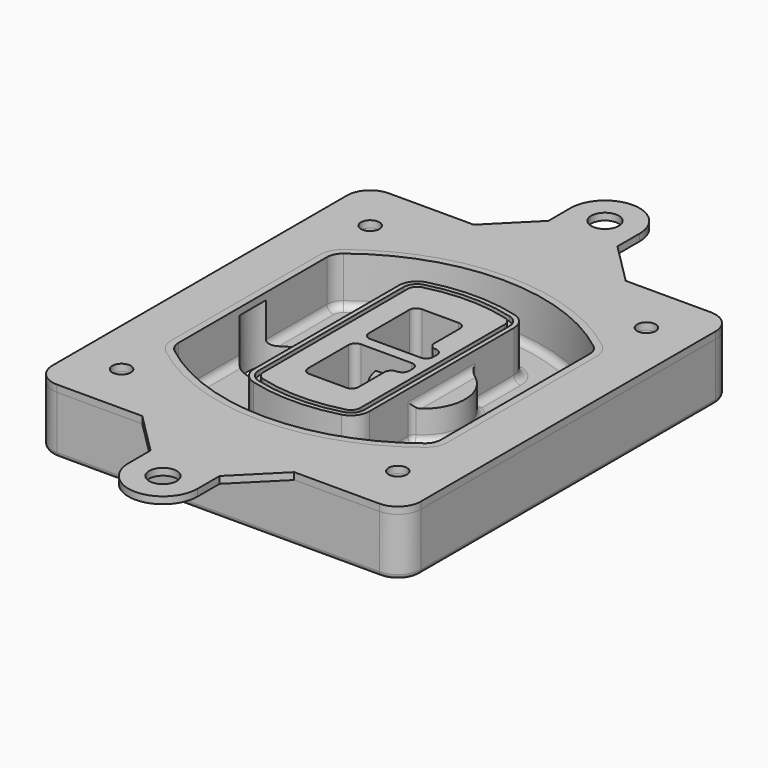
from build123d import *

# Parameters (mm, degrees)
F0_R      = 4
F1_DEPTH  = 25
F2_DEPTH  = 3
F3_DEPTH  = 18
F5_DEPTH  = 21
F6_DEPTH  = 2
F8_DEPTH  = 20
F9_DEPTH  = 16
F10_DEPTH = 25
F7_R      = 6
F7_R_2    = 4
F11_DEPTH = 6
F13_DEPTH = 9
F14_R     = 3
F15_R     = 2
F16_R     = 6
F16_R_2   = 4
F17_DEPTH = 3


with BuildPart() as f1:
    # F0 (on Top) → F1 (new body)
    with BuildSketch(Plane.XY):
        with BuildLine():
            ThreePointArc((-80, -80), (-77.0710678119, -87.0710678119), (-70, -90))
            Line((-70, -90), (70, -90))
            ThreePointArc((70, -90), (77.0710678119, -87.0710678119), (80, -80))
            Line((80, -80), (80, 80))
            ThreePointArc((80, 80), (77.0710678119, 87.0710678119), (70, 90))
            Line((70, 90), (-70, 90))
            ThreePointArc((-70, 90), (-77.0710678119, 87.0710678119), (-80, 80))
            Line((-80, 80), (-80, -80))
        make_face()
        with Locations((-60, -67.5)):
            Circle(F0_R, mode=Mode.SUBTRACT)
        with Locations((60, -67.5)):
            Circle(F0_R, mode=Mode.SUBTRACT)
        with Locations((-60, 67.5)):
            Circle(F0_R, mode=Mode.SUBTRACT)
        with BuildLine():
            ThreePointArc((-64, 40.2934422872), (-62.5820384798, 46.4328484224), (-58.6153846154, 51.3286200352))
            ThreePointArc((-58.6153846154, 51.3286200352), (0, 71.5), (58.6153846154, 51.3286200352))
            ThreePointArc((58.6153846154, 51.3286200352), (62.5820384798, 46.4328484224), (64, 40.2934422872))
            Line((64, 40.2934422872), (64, -40.2934422872))
            ThreePointArc((64, -40.2934422872), (62.5820384798, -46.4328484224), (58.6153846154, -51.3286200352))
            ThreePointArc((58.6153846154, -51.3286200352), (0, -71.5), (-58.6153846154, -51.3286200352))
            ThreePointArc((-58.6153846154, -51.3286200352), (-62.5820384798, -46.4328484224), (-64, -40.2934422872))
            Line((-64, -40.2934422872), (-64, 40.2934422872))
        make_face(mode=Mode.SUBTRACT)
        with Locations((60, 67.5)):
            Circle(F0_R, mode=Mode.SUBTRACT)
        with BuildLine():
            ThreePointArc((58.6153846154, 51.3286200352), (0, 71.5), (-58.6153846154, 51.3286200352))
            ThreePointArc((-58.6153846154, 51.3286200352), (-62.5820384798, 46.4328484224), (-64, 40.2934422872))
            Line((-64, 40.2934422872), (-64, -40.2934422872))
            ThreePointArc((-64, -40.2934422872), (-62.5820384798, -46.4328484224), (-58.6153846154, -51.3286200352))
            ThreePointArc((-58.6153846154, -51.3286200352), (0, -71.5), (58.6153846154, -51.3286200352))
            ThreePointArc((58.6153846154, -51.3286200352), (62.5820384798, -46.4328484224), (64, -40.2934422872))
            Line((64, -40.2934422872), (64, 40.2934422872))
            ThreePointArc((64, 40.2934422872), (62.5820384798, 46.4328484224), (58.6153846154, 51.3286200352))
        make_face()
        with BuildLine():
            Line((-60, -40.2934422872), (-60, 40.2934422872))
            ThreePointArc((-60, 40.2934422872), (-58.9871703427, 44.6787323838), (-56.1538461538, 48.1757121072))
            ThreePointArc((-56.1538461538, 48.1757121072), (0, 67.5), (56.1538461538, 48.1757121072))
            ThreePointArc((56.1538461538, 48.1757121072), (58.9871703427, 44.6787323838), (60, 40.2934422872))
            Line((60, 40.2934422872), (60, -40.2934422872))
            ThreePointArc((60, -40.2934422872), (58.9871703427, -44.6787323838), (56.1538461538, -48.1757121072))
            ThreePointArc((56.1538461538, -48.1757121072), (0, -67.5), (-56.1538461538, -48.1757121072))
            ThreePointArc((-56.1538461538, -48.1757121072), (-58.9871703427, -44.6787323838), (-60, -40.2934422872))
        make_face(mode=Mode.SUBTRACT)
        with BuildLine():
            ThreePointArc((-56.1538461538, 48.1757121072), (-58.9871703427, 44.6787323838), (-60, 40.2934422872))
            Line((-60, 40.2934422872), (-60, -40.2934422872))
            ThreePointArc((-60, -40.2934422872), (-58.9871703427, -44.6787323838), (-56.1538461538, -48.1757121072))
            ThreePointArc((-56.1538461538, -48.1757121072), (0, -67.5), (56.1538461538, -48.1757121072))
            ThreePointArc((56.1538461538, -48.1757121072), (58.9871703427, -44.6787323838), (60, -40.2934422872))
            Line((60, -40.2934422872), (60, 40.2934422872))
            ThreePointArc((60, 40.2934422872), (58.9871703427, 44.6787323838), (56.1538461538, 48.1757121072))
            ThreePointArc((56.1538461538, 48.1757121072), (0, 67.5), (-56.1538461538, 48.1757121072))
        make_face()
        with BuildLine():
            ThreePointArc((54.3076923077, 45.8110311612), (56.2910192399, 43.3631453548), (57, 40.2934422872))
            Line((57, 40.2934422872), (57, -40.2934422872))
            ThreePointArc((57, -40.2934422872), (56.2910192399, -43.3631453548), (54.3076923077, -45.8110311612))
            ThreePointArc((54.3076923077, -45.8110311612), (0, -64.5), (-54.3076923077, -45.8110311612))
            ThreePointArc((-54.3076923077, -45.8110311612), (-56.2910192399, -43.3631453548), (-57, -40.2934422872))
            Line((-57, -40.2934422872), (-57, 40.2934422872))
            ThreePointArc((-57, 40.2934422872), (-56.2910192399, 43.3631453548), (-54.3076923077, 45.8110311612))
            ThreePointArc((-54.3076923077, 45.8110311612), (0, 64.5), (54.3076923077, 45.8110311612))
        make_face(mode=Mode.SUBTRACT)
        with BuildLine():
            Line((57, -40.2934422872), (57, 40.2934422872))
            ThreePointArc((57, 40.2934422872), (56.2910192399, 43.3631453548), (54.3076923077, 45.8110311612))
            ThreePointArc((54.3076923077, 45.8110311612), (0, 64.5), (-54.3076923077, 45.8110311612))
            ThreePointArc((-54.3076923077, 45.8110311612), (-56.2910192399, 43.3631453548), (-57, 40.2934422872))
            Line((-57, 40.2934422872), (-57, -40.2934422872))
            ThreePointArc((-57, -40.2934422872), (-56.2910192399, -43.3631453548), (-54.3076923077, -45.8110311612))
            ThreePointArc((-54.3076923077, -45.8110311612), (0, -64.5), (54.3076923077, -45.8110311612))
            ThreePointArc((54.3076923077, -45.8110311612), (56.2910192399, -43.3631453548), (57, -40.2934422872))
        make_face()
    extrude(amount=-F1_DEPTH)

    # F0 (on Top) → F2 (join)
    with BuildSketch(Plane.XY):
        with BuildLine():
            ThreePointArc((-56.1538461538, 48.1757121072), (-58.9871703427, 44.6787323838), (-60, 40.2934422872))
            Line((-60, 40.2934422872), (-60, -40.2934422872))
            ThreePointArc((-60, -40.2934422872), (-58.9871703427, -44.6787323838), (-56.1538461538, -48.1757121072))
            ThreePointArc((-56.1538461538, -48.1757121072), (0, -67.5), (56.1538461538, -48.1757121072))
            ThreePointArc((56.1538461538, -48.1757121072), (58.9871703427, -44.6787323838), (60, -40.2934422872))
            Line((60, -40.2934422872), (60, 40.2934422872))
            ThreePointArc((60, 40.2934422872), (58.9871703427, 44.6787323838), (56.1538461538, 48.1757121072))
            ThreePointArc((56.1538461538, 48.1757121072), (0, 67.5), (-56.1538461538, 48.1757121072))
        make_face()
        with BuildLine():
            ThreePointArc((54.3076923077, 45.8110311612), (56.2910192399, 43.3631453548), (57, 40.2934422872))
            Line((57, 40.2934422872), (57, -40.2934422872))
            ThreePointArc((57, -40.2934422872), (56.2910192399, -43.3631453548), (54.3076923077, -45.8110311612))
            ThreePointArc((54.3076923077, -45.8110311612), (0, -64.5), (-54.3076923077, -45.8110311612))
            ThreePointArc((-54.3076923077, -45.8110311612), (-56.2910192399, -43.3631453548), (-57, -40.2934422872))
            Line((-57, -40.2934422872), (-57, 40.2934422872))
            ThreePointArc((-57, 40.2934422872), (-56.2910192399, 43.3631453548), (-54.3076923077, 45.8110311612))
            ThreePointArc((-54.3076923077, 45.8110311612), (0, 64.5), (54.3076923077, 45.8110311612))
        make_face(mode=Mode.SUBTRACT)
    extrude(amount=F2_DEPTH)

    # F0 (on Top) → F3 (cut)
    with BuildSketch(Plane.XY):
        with BuildLine():
            Line((57, -40.2934422872), (57, 40.2934422872))
            ThreePointArc((57, 40.2934422872), (56.2910192399, 43.3631453548), (54.3076923077, 45.8110311612))
            ThreePointArc((54.3076923077, 45.8110311612), (0, 64.5), (-54.3076923077, 45.8110311612))
            ThreePointArc((-54.3076923077, 45.8110311612), (-56.2910192399, 43.3631453548), (-57, 40.2934422872))
            Line((-57, 40.2934422872), (-57, -40.2934422872))
            ThreePointArc((-57, -40.2934422872), (-56.2910192399, -43.3631453548), (-54.3076923077, -45.8110311612))
            ThreePointArc((-54.3076923077, -45.8110311612), (0, -64.5), (54.3076923077, -45.8110311612))
            ThreePointArc((54.3076923077, -45.8110311612), (56.2910192399, -43.3631453548), (57, -40.2934422872))
        make_face()
    extrude(amount=-F3_DEPTH, mode=Mode.SUBTRACT)

    # F4 (on face) → F5 (join, through all)
    with BuildSketch(Plane.XY.offset(3)):
        with BuildLine():
            ThreePointArc((-25, -39.2465276821), (-23.3511545998, -44.1109737193), (-19.0842911877, -46.9702398883))
            ThreePointArc((-19.0842911877, -46.9702398883), (0, -49.5), (19.0842911877, -46.9702398883))
            ThreePointArc((19.0842911877, -46.9702398883), (23.3511545998, -44.1109737193), (25, -39.2465276821))
            Line((25, -39.2465276821), (25, 39.2465276821))
            ThreePointArc((25, 39.2465276821), (23.3511545998, 44.1109737193), (19.0842911877, 46.9702398883))
            ThreePointArc((19.0842911877, 46.9702398883), (0, 49.5), (-19.0842911877, 46.9702398883))
            ThreePointArc((-19.0842911877, 46.9702398883), (-23.3511545998, 44.1109737193), (-25, 39.2465276821))
            Line((-25, 39.2465276821), (-25, -39.2465276821))
        make_face()
        with BuildLine():
            ThreePointArc((18.5632183908, 45.0393118368), (21.7633659499, 42.89486221), (23, 39.2465276821))
            Line((23, 39.2465276821), (23, -39.2465276821))
            ThreePointArc((23, -39.2465276821), (21.7633659499, -42.89486221), (18.5632183908, -45.0393118368))
            ThreePointArc((18.5632183908, -45.0393118368), (0, -47.5), (-18.5632183908, -45.0393118368))
            ThreePointArc((-18.5632183908, -45.0393118368), (-21.7633659499, -42.89486221), (-23, -39.2465276821))
            Line((-23, -39.2465276821), (-23, 39.2465276821))
            ThreePointArc((-23, 39.2465276821), (-21.7633659499, 42.89486221), (-18.5632183908, 45.0393118368))
            ThreePointArc((-18.5632183908, 45.0393118368), (0, 47.5), (18.5632183908, 45.0393118368))
        make_face(mode=Mode.SUBTRACT)
        with BuildLine():
            Line((23, -39.2465276821), (23, 39.2465276821))
            ThreePointArc((23, 39.2465276821), (21.7633659499, 42.89486221), (18.5632183908, 45.0393118368))
            ThreePointArc((18.5632183908, 45.0393118368), (0, 47.5), (-18.5632183908, 45.0393118368))
            ThreePointArc((-18.5632183908, 45.0393118368), (-21.7633659499, 42.89486221), (-23, 39.2465276821))
            Line((-23, 39.2465276821), (-23, -39.2465276821))
            ThreePointArc((-23, -39.2465276821), (-21.7633659499, -42.89486221), (-18.5632183908, -45.0393118368))
            ThreePointArc((-18.5632183908, -45.0393118368), (0, -47.5), (18.5632183908, -45.0393118368))
            ThreePointArc((18.5632183908, -45.0393118368), (21.7633659499, -42.89486221), (23, -39.2465276821))
        make_face()
        with BuildLine():
            ThreePointArc((18.0421455939, 43.1083837852), (20.1755772999, 41.6787507007), (21, 39.2465276821))
            Line((21, 39.2465276821), (21, -39.2465276821))
            ThreePointArc((21, -39.2465276821), (20.1755772999, -41.6787507007), (18.0421455939, -43.1083837852))
            ThreePointArc((18.0421455939, -43.1083837852), (0, -45.5), (-18.0421455939, -43.1083837852))
            ThreePointArc((-18.0421455939, -43.1083837852), (-20.1755772999, -41.6787507007), (-21, -39.2465276821))
            Line((-21, -39.2465276821), (-21, 39.2465276821))
            ThreePointArc((-21, 39.2465276821), (-20.1755772999, 41.6787507007), (-18.0421455939, 43.1083837852))
            ThreePointArc((-18.0421455939, 43.1083837852), (0, 45.5), (18.0421455939, 43.1083837852))
        make_face(mode=Mode.SUBTRACT)
        with BuildLine():
            Line((21, -39.2465276821), (21, 39.2465276821))
            ThreePointArc((21, 39.2465276821), (20.1755772999, 41.6787507007), (18.0421455939, 43.1083837852))
            ThreePointArc((18.0421455939, 43.1083837852), (0, 45.5), (-18.0421455939, 43.1083837852))
            ThreePointArc((-18.0421455939, 43.1083837852), (-20.1755772999, 41.6787507007), (-21, 39.2465276821))
            Line((-21, 39.2465276821), (-21, -39.2465276821))
            ThreePointArc((-21, -39.2465276821), (-20.1755772999, -41.6787507007), (-18.0421455939, -43.1083837852))
            ThreePointArc((-18.0421455939, -43.1083837852), (0, -45.5), (18.0421455939, -43.1083837852))
            ThreePointArc((18.0421455939, -43.1083837852), (20.1755772999, -41.6787507007), (21, -39.2465276821))
        make_face()
        with BuildLine():
            Line((-8, -2.5), (14, -2.5))
            ThreePointArc((14, -2.5), (16.1213203436, -3.3786796564), (17, -5.5))
            Line((17, -5.5), (17, -7.5))
            ThreePointArc((17, -7.5), (16.1213203436, -9.6213203436), (14, -10.5))
            ThreePointArc((14, -10.5), (11.8786796564, -11.3786796564), (11, -13.5))
            Line((11, -13.5), (11, -27.5))
            ThreePointArc((11, -27.5), (10.1213203436, -29.6213203436), (8, -30.5))
            Line((8, -30.5), (-8, -30.5))
            ThreePointArc((-8, -30.5), (-10.1213203436, -29.6213203436), (-11, -27.5))
            Line((-11, -27.5), (-11, -5.5))
            ThreePointArc((-11, -5.5), (-10.1213203436, -3.3786796564), (-8, -2.5))
        make_face(mode=Mode.SUBTRACT)
        with BuildLine():
            ThreePointArc((-8, 2.5), (-10.1213203436, 3.3786796564), (-11, 5.5))
            Line((-11, 5.5), (-11, 27.5))
            ThreePointArc((-11, 27.5), (-10.1213203436, 29.6213203436), (-8, 30.5))
            Line((-8, 30.5), (8, 30.5))
            ThreePointArc((8, 30.5), (10.1213203436, 29.6213203436), (11, 27.5))
            Line((11, 27.5), (11, 13.5))
            ThreePointArc((11, 13.5), (11.8786796564, 11.3786796564), (14, 10.5))
            ThreePointArc((14, 10.5), (16.1213203436, 9.6213203436), (17, 7.5))
            Line((17, 7.5), (17, 5.5))
            ThreePointArc((17, 5.5), (16.1213203436, 3.3786796564), (14, 2.5))
            Line((14, 2.5), (-8, 2.5))
        make_face(mode=Mode.SUBTRACT)
    extrude(amount=-F5_DEPTH)

    # F4 (on face) → F6 (cut)
    with BuildSketch(Plane.XY.offset(3)):
        with BuildLine():
            Line((23, -39.2465276821), (23, 39.2465276821))
            ThreePointArc((23, 39.2465276821), (21.7633659499, 42.89486221), (18.5632183908, 45.0393118368))
            ThreePointArc((18.5632183908, 45.0393118368), (0, 47.5), (-18.5632183908, 45.0393118368))
            ThreePointArc((-18.5632183908, 45.0393118368), (-21.7633659499, 42.89486221), (-23, 39.2465276821))
            Line((-23, 39.2465276821), (-23, -39.2465276821))
            ThreePointArc((-23, -39.2465276821), (-21.7633659499, -42.89486221), (-18.5632183908, -45.0393118368))
            ThreePointArc((-18.5632183908, -45.0393118368), (0, -47.5), (18.5632183908, -45.0393118368))
            ThreePointArc((18.5632183908, -45.0393118368), (21.7633659499, -42.89486221), (23, -39.2465276821))
        make_face()
        with BuildLine():
            ThreePointArc((18.0421455939, 43.1083837852), (20.1755772999, 41.6787507007), (21, 39.2465276821))
            Line((21, 39.2465276821), (21, -39.2465276821))
            ThreePointArc((21, -39.2465276821), (20.1755772999, -41.6787507007), (18.0421455939, -43.1083837852))
            ThreePointArc((18.0421455939, -43.1083837852), (0, -45.5), (-18.0421455939, -43.1083837852))
            ThreePointArc((-18.0421455939, -43.1083837852), (-20.1755772999, -41.6787507007), (-21, -39.2465276821))
            Line((-21, -39.2465276821), (-21, 39.2465276821))
            ThreePointArc((-21, 39.2465276821), (-20.1755772999, 41.6787507007), (-18.0421455939, 43.1083837852))
            ThreePointArc((-18.0421455939, 43.1083837852), (0, 45.5), (18.0421455939, 43.1083837852))
        make_face(mode=Mode.SUBTRACT)
    extrude(amount=-F6_DEPTH, mode=Mode.SUBTRACT)

    # F7 (on face) → F8 (join)
    with BuildSketch(Plane(origin=(0, 0, -25), x_dir=(1, 0, 0), z_dir=(0, 0, -1))):
        with BuildLine():
            ThreePointArc((3.28842436, 0), (16.7567035675, 13.4682792075), (30.224982775, 0))
            Line((30.224982775, 0), (35.224982775, 0))
            ThreePointArc((35.224982775, 0), (16.7567035675, 18.4682792075), (-1.71157564, 0))
            Line((-1.71157564, 0), (3.28842436, 0))
        make_face()
        with BuildLine():
            Line((3.28842436, 0), (30.224982775, 0))
            ThreePointArc((30.224982775, 0), (16.7567035675, 13.4682792075), (3.28842436, 0))
        make_face()
        with BuildLine():
            ThreePointArc((3.28842436, 0), (16.7567035675, -13.4682792075), (30.224982775, 0))
            Line((30.224982775, 0), (3.28842436, 0))
        make_face()
        with BuildLine():
            Line((35.224982775, 0), (30.224982775, 0))
            ThreePointArc((30.224982775, 0), (16.7567035675, -13.4682792075), (3.28842436, 0))
            Line((3.28842436, 0), (-1.71157564, 0))
            ThreePointArc((-1.71157564, 0), (16.7567035675, -18.4682792075), (35.224982775, 0))
        make_face()
    extrude(amount=-F8_DEPTH)

    # F7 (on face) → F9 (cut)
    with BuildSketch(Plane(origin=(0, 0, -25), x_dir=(1, 0, 0), z_dir=(0, 0, -1))):
        with BuildLine():
            Line((3.28842436, 0), (30.224982775, 0))
            ThreePointArc((30.224982775, 0), (16.7567035675, 13.4682792075), (3.28842436, 0))
        make_face()
        with BuildLine():
            ThreePointArc((3.28842436, 0), (16.7567035675, -13.4682792075), (30.224982775, 0))
            Line((30.224982775, 0), (3.28842436, 0))
        make_face()
    extrude(amount=-F9_DEPTH, mode=Mode.SUBTRACT)

    # F7 (on face) → F10 (cut)
    with BuildSketch(Plane(origin=(0, 0, -25), x_dir=(1, 0, 0), z_dir=(0, 0, -1))):
        with BuildLine():
            Line((-59.0318229325, 0), (-32.0952645175, 0))
            ThreePointArc((-32.0952645175, 0), (-45.563543725, 13.4682792075), (-59.0318229325, 0))
        make_face()
        with BuildLine():
            ThreePointArc((-59.0318229325, 0), (-45.563543725, -13.4682792075), (-32.0952645175, 0))
            Line((-32.0952645175, 0), (-59.0318229325, 0))
        make_face()
    extrude(amount=-F10_DEPTH, mode=Mode.SUBTRACT)

    # F7 (on face) → F11 (cut)
    with BuildSketch(Plane(origin=(0, 0, -25), x_dir=(1, 0, 0), z_dir=(0, 0, -1))):
        with Locations((60, -67.5)):
            Circle(F7_R)
        with Locations((60, -67.5)):
            Circle(F7_R_2, mode=Mode.SUBTRACT)
        with Locations((-60, -67.5)):
            Circle(F7_R)
        with Locations((-60, -67.5)):
            Circle(F7_R_2, mode=Mode.SUBTRACT)
        with Locations((-60, 67.5)):
            Circle(F7_R)
        with Locations((-60, 67.5)):
            Circle(F7_R_2, mode=Mode.SUBTRACT)
        with Locations((60, 67.5)):
            Circle(F7_R)
        with Locations((60, 67.5)):
            Circle(F7_R_2, mode=Mode.SUBTRACT)
    extrude(amount=-F11_DEPTH, mode=Mode.SUBTRACT)

    # F12 (on face) → F13 (cut, through all)
    with BuildSketch(Plane(origin=(0, 0, -9), x_dir=(1, 0, 0), z_dir=(0, 0, -1))):
        with BuildLine():
            Line((11, 13.5), (11, 17.5481537753))
            ThreePointArc((11, 17.5481537753), (2.5696536419, 11.8239143813), (-1.5415842455, 2.5))
            Line((-1.5415842455, 2.5), (3.5224848595, 2.5))
            ThreePointArc((3.5224848595, 2.5), (6.1857188154, 8.3455872281), (11.2536447004, 12.2927168648))
            ThreePointArc((11.2536447004, 12.2927168648), (11.0640958889, 12.8831798879), (11, 13.5))
        make_face()
        with BuildLine():
            ThreePointArc((11.2536447004, -12.2927168648), (6.1857188154, -8.3455872281), (3.5224848595, -2.5))
            Line((3.5224848595, -2.5), (-1.5415842455, -2.5))
            ThreePointArc((-1.5415842455, -2.5), (2.5696536419, -11.8239143813), (11, -17.5481537753))
            Line((11, -17.5481537753), (11, -13.5))
            ThreePointArc((11, -13.5), (11.0640958889, -12.8831798879), (11.2536447004, -12.2927168648))
        make_face()
        with BuildLine():
            ThreePointArc((11.2536447004, 12.2927168648), (6.1857188154, 8.3455872281), (3.5224848595, 2.5))
            Line((3.5224848595, 2.5), (14, 2.5))
            ThreePointArc((14, 2.5), (16.1213203436, 3.3786796564), (17, 5.5))
            Line((17, 5.5), (17, 7.5))
            ThreePointArc((17, 7.5), (16.1213203436, 9.6213203436), (14, 10.5))
            ThreePointArc((14, 10.5), (12.3601599782, 10.9878446101), (11.2536447004, 12.2927168648))
        make_face()
        with BuildLine():
            Line((14, -2.5), (3.5224848595, -2.5))
            ThreePointArc((3.5224848595, -2.5), (6.1857188154, -8.3455872281), (11.2536447004, -12.2927168648))
            ThreePointArc((11.2536447004, -12.2927168648), (12.3601599782, -10.9878446101), (14, -10.5))
            ThreePointArc((14, -10.5), (16.1213203436, -9.6213203436), (17, -7.5))
            Line((17, -7.5), (17, -5.5))
            ThreePointArc((17, -5.5), (16.1213203436, -3.3786796564), (14, -2.5))
        make_face()
    extrude(amount=F13_DEPTH, mode=Mode.SUBTRACT)

    # F14
    f14_edges = [f1.edges().sort_by_distance(p)[0] for p in [
        (-57, -23.703476, -18),
        (-57, 23.703476, -18),
        (25, 0, -5),
        (25, 16.526506, -11.5),
        (25, -16.526506, -11.5),
        (25, -27.886517, -18),
        (35.224983, 0, -18),
    ]]
    fillet(f14_edges, radius=F14_R)

    # F15
    f15_edges = [f1.edges().sort_by_distance(p)[0] for p in [
        (0, -90, -25),
    ]]
    fillet(f15_edges, radius=F15_R)


with BuildPart() as f17:
    # F16 (on face) → F17 (new body, through all)
    with BuildSketch(Plane.XY):
        with BuildLine():
            Line((-33, 90), (33, 90))
            Line((33, 90), (15, 108))
            Line((15, 108), (15, 120))
            ThreePointArc((15, 120), (0, 135), (-15, 120))
            Line((-15, 120), (-15, 108))
            Line((-15, 108), (-33, 90))
        make_face()
        with Locations((0, 120)):
            Circle(F16_R, mode=Mode.SUBTRACT)
        with BuildLine():
            ThreePointArc((70, -90), (77.0710678119, -87.0710678119), (80, -80))
            Line((80, -80), (80, 80))
            ThreePointArc((80, 80), (77.0710678119, 87.0710678119), (70, 90))
            Line((70, 90), (33, 90))
            Line((33, 90), (-33, 90))
            Line((-33, 90), (-70, 90))
            ThreePointArc((-70, 90), (-77.0710678119, 87.0710678119), (-80, 80))
            Line((-80, 80), (-80, -80))
            ThreePointArc((-80, -80), (-77.0710678119, -87.0710678119), (-70, -90))
            Line((-70, -90), (-33, -90))
            Line((-33, -90), (33, -90))
            Line((33, -90), (70, -90))
        make_face()
        with Locations((-60, -67.5)):
            Circle(F16_R_2, mode=Mode.SUBTRACT)
        with Locations((60, -67.5)):
            Circle(F16_R_2, mode=Mode.SUBTRACT)
        with Locations((-60, 67.5)):
            Circle(F16_R_2, mode=Mode.SUBTRACT)
        with BuildLine():
            ThreePointArc((56.1538461538, -48.1757121072), (0, -67.5), (-56.1538461538, -48.1757121072))
            ThreePointArc((-56.1538461538, -48.1757121072), (-58.9871703427, -44.6787323838), (-60, -40.2934422872))
            Line((-60, -40.2934422872), (-60, 40.2934422872))
            ThreePointArc((-60, 40.2934422872), (-58.9871703427, 44.6787323838), (-56.1538461538, 48.1757121072))
            ThreePointArc((-56.1538461538, 48.1757121072), (0, 67.5), (56.1538461538, 48.1757121072))
            ThreePointArc((56.1538461538, 48.1757121072), (58.9871703427, 44.6787323838), (60, 40.2934422872))
            Line((60, 40.2934422872), (60, -40.2934422872))
            ThreePointArc((60, -40.2934422872), (58.9871703427, -44.6787323838), (56.1538461538, -48.1757121072))
        make_face(mode=Mode.SUBTRACT)
        with Locations((60, 67.5)):
            Circle(F16_R_2, mode=Mode.SUBTRACT)
        with BuildLine():
            Line((15, -108), (33, -90))
            Line((33, -90), (-33, -90))
            Line((-33, -90), (-15, -108))
            Line((-15, -108), (-15, -120))
            ThreePointArc((-15, -120), (0, -135), (15, -120))
            Line((15, -120), (15, -108))
        make_face()
        with Locations((0, -120)):
            Circle(F16_R, mode=Mode.SUBTRACT)
    extrude(amount=F17_DEPTH)


solid = Compound([f1.part, f17.part])
